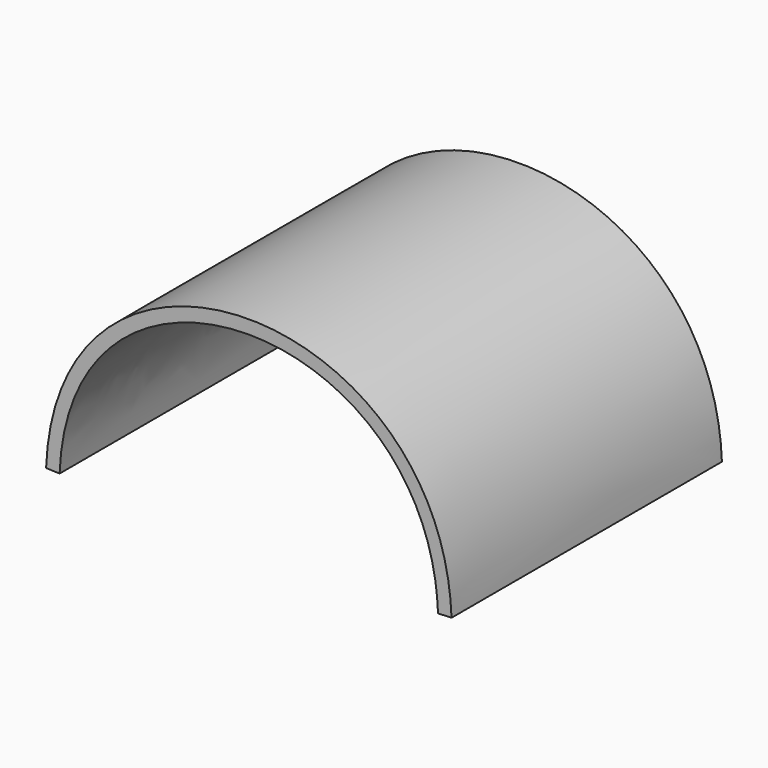
from build123d import *

# Parameters (mm, degrees)
F1_DEPTH = 25


with BuildPart() as f1:
    # F0 (on Front) → F1 (new body)
    with BuildSketch(Plane.XZ):
        with BuildLine():
            Line((-14.9963256411, 0.0382544926), (-13.9970576121, 0))
            add(Edge.make_bspline(
                [(-13.9970576121, 0), (-13.302341298, 18.1470921482), (13.302341298, 18.1470921482), (13.9970576121, 0)],
                knots=[0, 0, 0, 0, 27.9941152242, 27.9941152242, 27.9941152242, 27.9941152242], degree=3))
            Line((13.9970576121, 0), (14.9963256411, 0.0382544926))
            add(Edge.make_bspline(
                [(-14.9963256411, 0.0382544926), (-14.9048193337, 2.4285443973), (-13.8625817733, 6.6722308908), (-10.2984637837, 11.2723953851), (-5.4512440405, 14.0078344849), (0, 14.9115614242), (5.4512440405, 14.0078344849), (10.2984637837, 11.2723953851), (13.8625817733, 6.6722308908), (14.9048193337, 2.4285443973), (14.9963256411, 0.0382544926)],
                knots=[0, 0, 0, 0, 0.125, 0.25, 0.375, 0.5, 0.625, 0.75, 0.875, 1, 1, 1, 1], degree=3))
        make_face()
    extrude(amount=F1_DEPTH)


solid = f1.part
